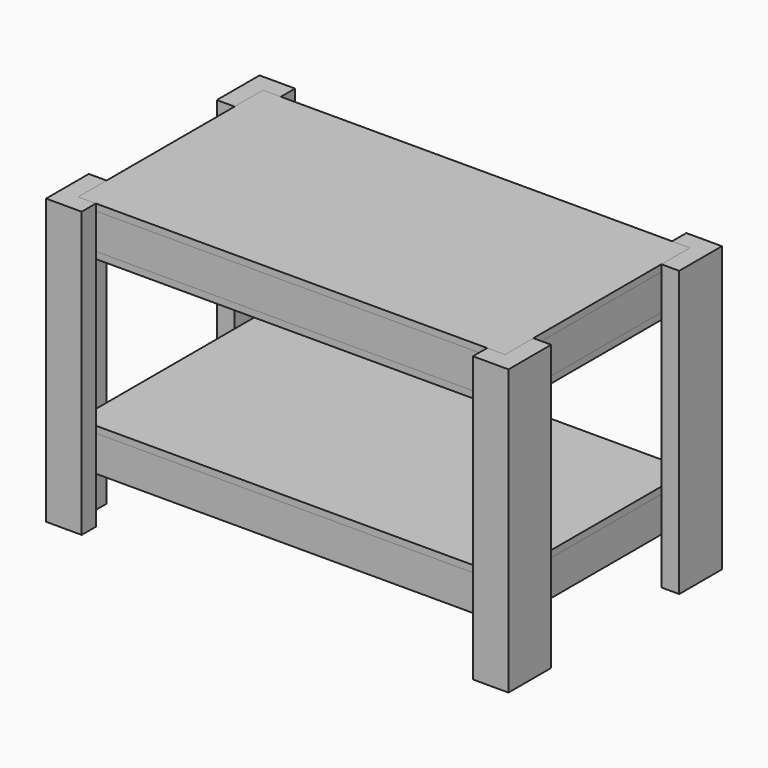
from build123d import *

# Parameters (mm, degrees)
F2_W     = 50.8
F2_H     = 101.6
F3_DEPTH = 812.8
F4_DEPTH = 19.05
F5_W     = 50.8
F5_H     = 558.8
F6_DEPTH = 101.6


# Not quite as in the source:
# - a length typed as a fraction of an inch, garbled in the dataset ("3 / 203.2 mm" for 3/8 in), is restored


with BuildPart() as f3:
    # F2 (on Top) → F3 (new body)
    with BuildSketch(Plane.XY):
        with Locations((-635, 279.4)):
            Rectangle(F2_W, F2_H)
        Polygon((-609.6, 330.2), (-558.8, 330.2), (-558.8, 381), (-660.4, 381), (-660.4, 330.2), align=None)
    extrude(amount=-F3_DEPTH)


with BuildPart() as f3b:
    # F2 (on Top) → F3, piece 2 (new body)
    with BuildSketch(Plane.XY):
        Polygon((558.8, 330.2), (609.6, 330.2), (660.4, 330.2), (660.4, 381), (558.8, 381), align=None)
        with Locations((635, 279.4)):
            Rectangle(F2_W, F2_H)
    extrude(amount=-F3_DEPTH)


with BuildPart() as f3c:
    # F2 (on Top) → F3, piece 3 (new body)
    with BuildSketch(Plane.XY):
        with Locations((635, -279.4)):
            Rectangle(F2_W, F2_H)
        Polygon((660.4, -330.2), (609.6, -330.2), (558.8, -330.2), (558.8, -381), (660.4, -381), align=None)
    extrude(amount=-F3_DEPTH)


with BuildPart() as f3d:
    # F2 (on Top) → F3, piece 4 (new body)
    with BuildSketch(Plane.XY):
        with Locations((-635, -279.4)):
            Rectangle(F2_W, F2_H)
        Polygon((-558.8, -381), (-558.8, -330.2), (-609.6, -330.2), (-660.4, -330.2), (-660.4, -381), align=None)
    extrude(amount=-F3_DEPTH)


with BuildPart() as f4:
    # F2 (on Top) → F4 (new body)
    with BuildSketch(Plane.XY):
        Polygon((609.6, 228.6), (609.6, 330.2), (558.8, 330.2), (-558.8, 330.2), (-609.6, 330.2), (-609.6, 228.6), (-609.6, -228.6), (-609.6, -330.2), (-558.8, -330.2), (558.8, -330.2), (609.6, -330.2), (609.6, -228.6), align=None)
    extrude(amount=-F4_DEPTH)


with BuildPart() as f6:
    # F5 (on face) → F6 (new body)
    with BuildSketch(Plane(origin=(0, 0, -19.05), x_dir=(1, 0, 0), z_dir=(0, 0, -1))):
        Polygon((609.6, 330.2), (558.8, 330.2), (558.8, 279.4), (558.8, -279.4), (558.8, -330.2), (609.6, -330.2), align=None)
        Polygon((-558.8, -279.4), (-558.8, -330.2), (558.8, -330.2), (558.8, -279.4), (220.1333333333, -279.4), (169.3333333333, -279.4), (-169.3333333333, -279.4), (-220.1333333333, -279.4), align=None)
        Polygon((-558.8, 330.2), (-609.6, 330.2), (-609.6, -330.2), (-558.8, -330.2), (-558.8, -279.4), (-558.8, 279.4), align=None)
        with Locations((194.7333333333, 0)):
            Rectangle(F5_W, F5_H)
        with Locations((-194.7333333333, 0)):
            Rectangle(F5_W, F5_H)
        Polygon((558.8, 330.2), (-558.8, 330.2), (-558.8, 279.4), (-220.1333333333, 279.4), (-169.3333333333, 279.4), (169.3333333333, 279.4), (220.1333333333, 279.4), (558.8, 279.4), align=None)
    extrude(amount=F6_DEPTH)


with BuildPart() as f7_1:
    # F7: copy of F4
    add(f4.part.moved(Location((0, 0, -120.65))))


with BuildPart() as f8_1:
    # F8: copy of F6
    add(f6.part.moved(Location((0, 0, -558.8))))


with BuildPart() as f8_2:
    # F8: copy of F4
    add(f4.part.moved(Location((0, 0, -558.8))))


solid = Compound([f3.part, f3b.part, f3c.part, f3d.part, f4.part, f6.part, f7_1.part, f8_1.part, f8_2.part])
